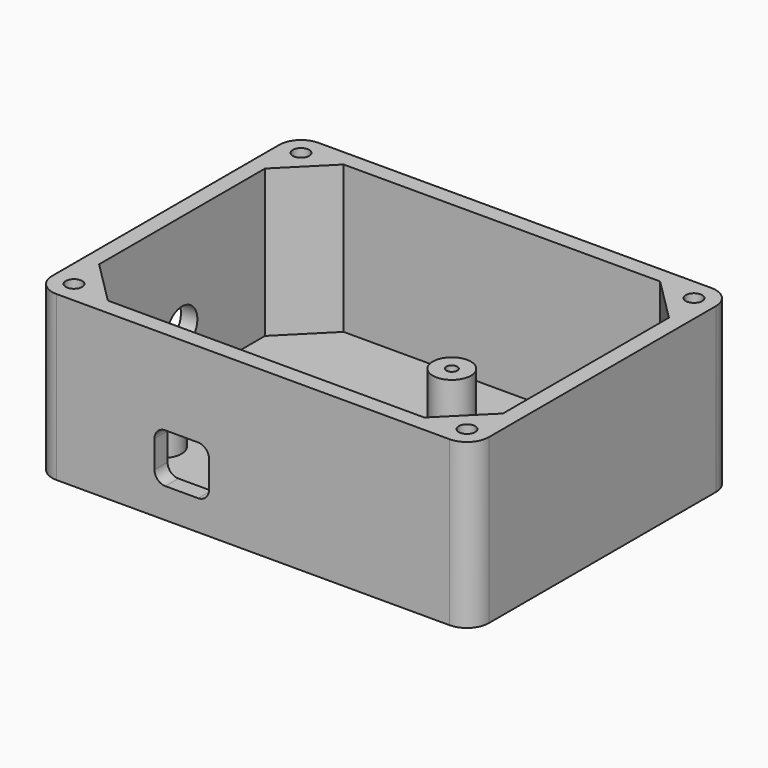
from build123d import *

# Parameters (mm, degrees)
F0_W      = 101.6
F0_H      = 76.2
F1_DEPTH  = 38.1
F2_T      = -3.81
F3_SIZE   = 10.16
F4_R      = 4.445
F4_R_2    = 1.27
F6_DEPTH  = 11.43
F5_R      = 4.445
F7_DEPTH  = 3.81
F8_W      = 12.7
F8_H      = 11.43
F9_DEPTH  = 3.81
F10_R     = 2.54
F11_R     = 5.08
F12_R     = 1.905
F13_DEPTH = 16.51


with BuildPart() as f1:
    # F0 (on Top) → F1 (new body)
    with BuildSketch(Plane.XY):
        with Locations((1.9488222897, 0.8362135466)):
            Rectangle(F0_W, F0_H)
    extrude(amount=F1_DEPTH)

    # F2
    f2_openings = [f1.faces().sort_by_distance(p)[0] for p in [
        (1.948822, 0.836214, 38.1),
    ]]
    offset(amount=F2_T, openings=f2_openings)

    # F3
    f3_edges = [f1.edges().sort_by_distance(p)[0] for p in [
        (-45.041178, 35.126214, 20.955),
        (48.938822, 35.126214, 20.955),
        (48.938822, -33.453786, 20.955),
        (-45.041178, -33.453786, 20.955),
    ]]
    chamfer(f3_edges, length=F3_SIZE)

    # F4 (on face) → F6 (join)
    with BuildSketch(Plane.XY.offset(3.81)):
        with Locations((-32.3411777103, -20.7537864534)):
            Circle(F4_R)
        with Locations((-32.3411777103, -20.7537864534)):
            Circle(F4_R_2, mode=Mode.SUBTRACT)
        with Locations((3.2188222897, 18.9762135466)):
            Circle(F4_R)
        with Locations((3.2188222897, 18.9762135466)):
            Circle(F4_R_2, mode=Mode.SUBTRACT)
    extrude(amount=F6_DEPTH)

    # F5 (on face) → F7 (cut, through all)
    with BuildSketch(Plane.YZ.offset(-45.0411777103)):
        with Locations((0.8362135466, 15.24)):
            Circle(F5_R)
    extrude(amount=-F7_DEPTH, mode=Mode.SUBTRACT)

    # F8 (on face) → F9 (cut, through all)
    with BuildSketch(Plane(origin=(0, -33.4537864534, 0), x_dir=(-1, 0, 0), z_dir=(0, 1, 0))):
        with Locations((14.6373170428, 12.7)):
            Rectangle(F8_W, F8_H)
    extrude(amount=-F9_DEPTH, mode=Mode.SUBTRACT)

    # F10
    f10_edges = [f1.edges().sort_by_distance(p)[0] for p in [
        (-8.287317, -35.358786, 6.985),
        (-20.987317, -35.358786, 6.985),
        (-20.987317, -35.358786, 18.415),
        (-8.287317, -35.358786, 18.415),
    ]]
    fillet(f10_edges, radius=F10_R)

    # F11
    f11_edges = [f1.edges().sort_by_distance(p)[0] for p in [
        (-48.851178, -37.263786, 19.05),
        (52.748822, -37.263786, 19.05),
        (52.748822, 38.936214, 19.05),
        (-48.851178, 38.936214, 19.05),
    ]]
    fillet(f11_edges, radius=F11_R)

    # F12 (on face) → F13 (cut)
    with BuildSketch(Plane.XY.offset(38.1)):
        with Locations((-43.7711777103, 33.8562135466)):
            Circle(F12_R)
        with Locations((-43.7711777103, -32.1837864534)):
            Circle(F12_R)
        with Locations((47.6688222897, 33.8562135466)):
            Circle(F12_R)
        with Locations((47.6688222897, -32.1837864534)):
            Circle(F12_R)
        with Locations((139.1088222897, 33.8562135466)):
            Circle(F12_R)
        with Locations((139.1088222897, -32.1837864534)):
            Circle(F12_R)
    extrude(amount=-F13_DEPTH, mode=Mode.SUBTRACT)


solid = f1.part
